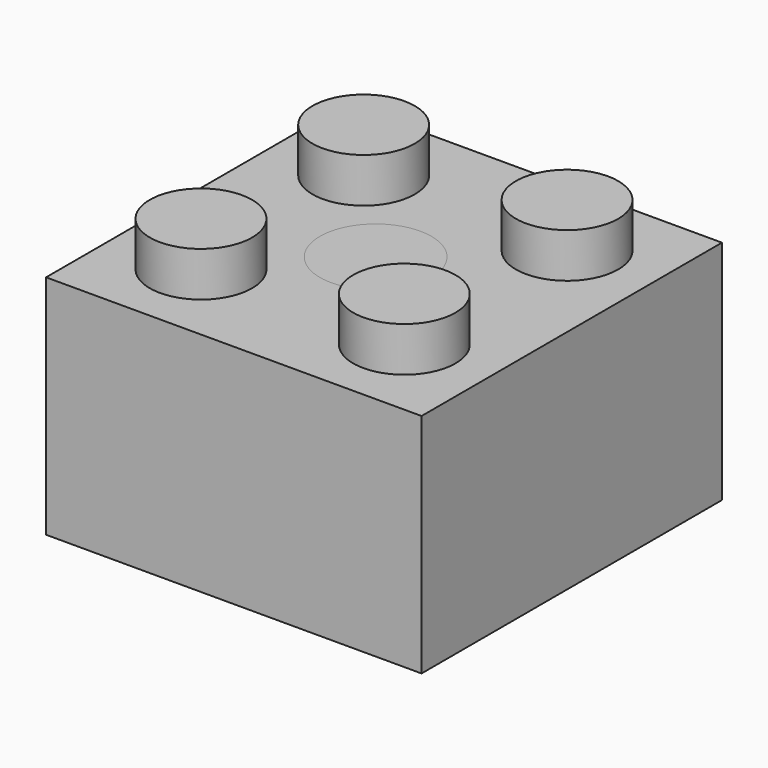
from build123d import *

# Parameters (mm, degrees)
F0_W     = 15.82
F0_H     = 15.82
F0_R     = 2.155
F0_R_2   = 2.35
F1_DEPTH = 9.55
F2_DEPTH = 1.88
F3_DEPTH = 4.88


with BuildPart() as f1:
    # F0 (on Top) → F1 (new body)
    with BuildSketch(Plane.XY):
        with Locations((0.3504429367, 0)):
            Rectangle(F0_W, F0_H)
        with Locations((-3.9345570633, -4.285)):
            Circle(F0_R, mode=Mode.SUBTRACT)
        Circle(F0_R_2, mode=Mode.SUBTRACT)
        with Locations((4.6354429367, -4.285)):
            Circle(F0_R, mode=Mode.SUBTRACT)
        with Locations((-3.9345570633, 4.285)):
            Circle(F0_R, mode=Mode.SUBTRACT)
        with Locations((4.6354429367, 4.285)):
            Circle(F0_R, mode=Mode.SUBTRACT)
        with Locations((-3.9345570633, -4.285)):
            Circle(F0_R)
        with Locations((-3.9345570633, 4.285)):
            Circle(F0_R)
        with Locations((4.6354429367, 4.285)):
            Circle(F0_R)
        with Locations((4.6354429367, -4.285)):
            Circle(F0_R)
    extrude(amount=-F1_DEPTH)

    # F0 (on Top) → F2 (join)
    with BuildSketch(Plane.XY):
        with Locations((-3.9345570633, 4.285)):
            Circle(F0_R)
        with Locations((-3.9345570633, -4.285)):
            Circle(F0_R)
        with Locations((4.6354429367, 4.285)):
            Circle(F0_R)
        with Locations((4.6354429367, -4.285)):
            Circle(F0_R)
    extrude(amount=F2_DEPTH)


with BuildPart() as f3:
    # F0 (on Top) → F3 (new body)
    with BuildSketch(Plane.XY):
        Circle(F0_R_2)
    extrude(amount=-F3_DEPTH)


solid = Compound([f1.part, f3.part])
